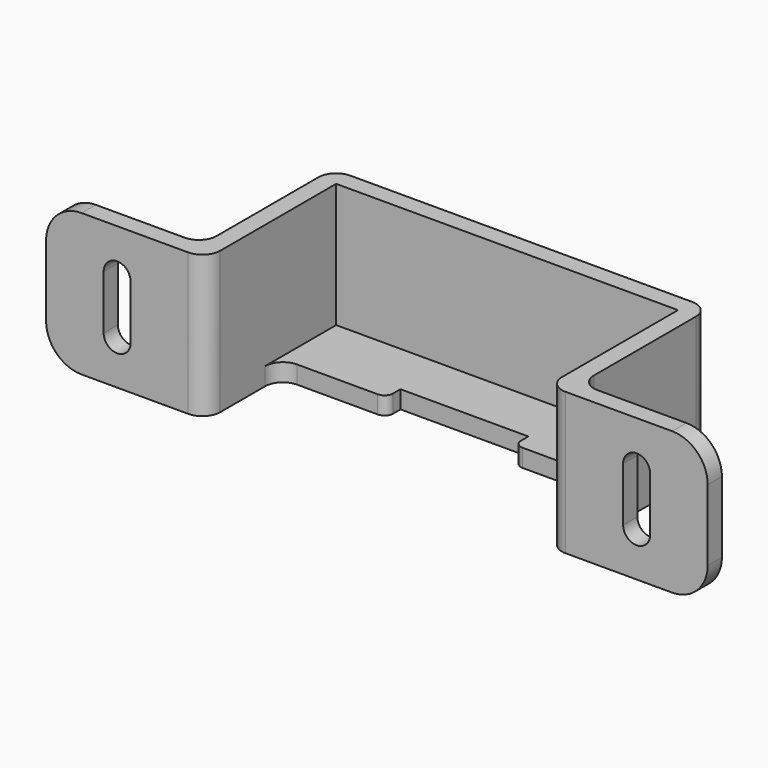
from build123d import *

# Parameters (mm, degrees)
F1_DEPTH  = 25.4
F2_R      = 3.175
F4_DEPTH  = 32.259
F5_R      = 6.35
F6_W      = 61.087
F6_H      = 12.7
F7_DEPTH  = 3.175
F8_R      = 3.175
F9_W      = 22.86
F9_H      = 3.175
F10_DEPTH = 25.4
F11_R     = 1.524


with BuildPart() as f1:
    # F0 (on Top) → F1 (new body)
    with BuildSketch(Plane.XY):
        Polygon((-30.5435, 29.083), (0, 29.083), (30.5435, 29.083), (30.5435, 0), (59.1185, 0), (59.1185, 3.175), (33.7185, 3.175), (33.7185, 32.258), (0, 32.258), (-33.7185, 32.258), (-33.7185, 3.175), (-59.1185, 3.175), (-59.1185, 0), (-30.5435, 0), align=None)
    extrude(amount=F1_DEPTH)

    # F2
    f2_edges = [f1.edges().sort_by_distance(p)[0] for p in [
        (-30.5435, 0, 12.7),
        (30.5435, 0, 12.7),
    ]]
    fillet(f2_edges, radius=F2_R)

    # F3 (on Front) → F4 (cut, through all)
    with BuildSketch(Plane.XZ):
        with BuildLine():
            ThreePointArc((-48.8315, 7.8105), (-46.4185, 5.3975), (-44.0055, 7.8105))
            Line((-44.0055, 7.8105), (-44.0055, 17.4625))
            ThreePointArc((-44.0055, 17.4625), (-46.4185, 19.8755), (-48.8315, 17.4625))
            Line((-48.8315, 17.4625), (-48.8315, 7.8105))
        make_face()
        with BuildLine():
            ThreePointArc((48.8315, 17.4498), (46.4185, 19.8628), (44.0055, 17.4498))
            Line((44.0055, 17.4498), (44.0055, 7.7978))
            ThreePointArc((44.0055, 7.7978), (46.4185, 5.3848), (48.8315, 7.7978))
            Line((48.8315, 7.7978), (48.8315, 17.4498))
        make_face()
    extrude(amount=-F4_DEPTH, mode=Mode.SUBTRACT)

    # F5
    f5_edges = [f1.edges().sort_by_distance(p)[0] for p in [
        (-59.1185, 1.5875, 0),
        (-59.1185, 1.5875, 25.4),
        (59.1185, 1.5875, 25.4),
        (59.1185, 1.5875, 0),
    ]]
    fillet(f5_edges, radius=F5_R)

    # F6 (on face) → F7 (join)
    with BuildSketch(Plane(origin=(0, 0, 0), x_dir=(1, 0, 0), z_dir=(0, 0, -1))):
        with Locations((0, -22.733)):
            Rectangle(F6_W, F6_H)
    extrude(amount=-F7_DEPTH)

    # F8
    f8_edges = [f1.edges().sort_by_distance(p)[0] for p in [
        (33.7185, 3.175, 12.7),
        (33.7185, 32.258, 12.7),
        (-33.7185, 32.258, 12.7),
        (-33.7185, 3.175, 12.7),
        (30.5435, 16.383, 1.5875),
        (-30.5435, 16.383, 1.5875),
    ]]
    fillet(f8_edges, radius=F8_R)

    # F9 (on face) → F10 (cut)
    with BuildSketch(Plane.XY.offset(3.175)):
        with Locations((0, 17.9705)):
            Rectangle(F9_W, F9_H)
    extrude(amount=-F10_DEPTH, mode=Mode.SUBTRACT)

    # F11
    f11_edges = [f1.edges().sort_by_distance(p)[0] for p in [
        (-11.43, 16.383, 1.5875),
        (11.43, 16.383, 1.5875),
    ]]
    fillet(f11_edges, radius=F11_R)


solid = f1.part
